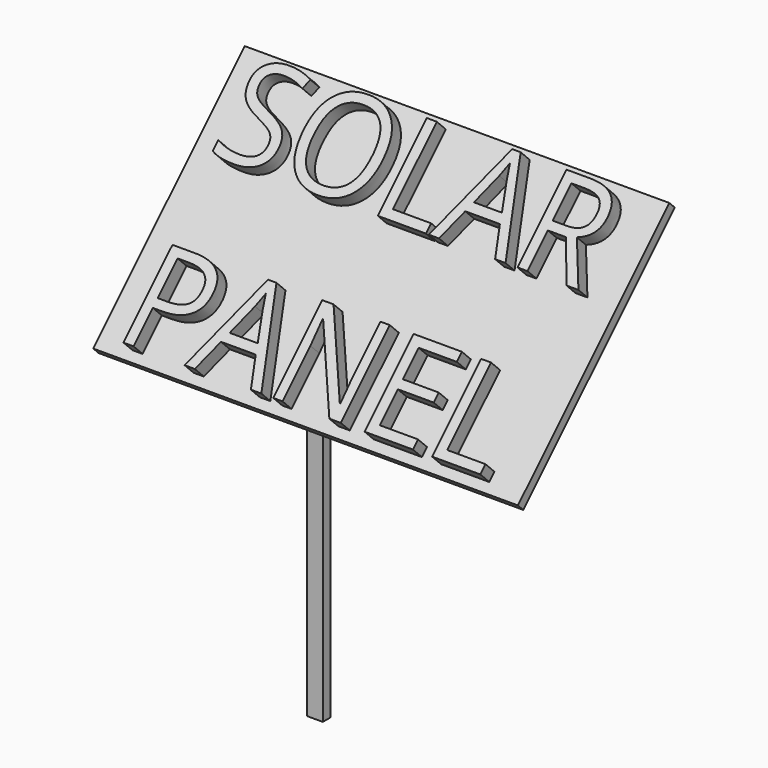
from build123d import *

# Parameters (mm, degrees)
F0_W         = 25
F0_H         = 396.1333930492
F1_DEPTH     = 15
F2_W         = 668.0434644222
F2_H         = 421.1661219597
F3_DEPTH     = 15
F4_TEXT_SIZE = 190.7505836769
F5_DEPTH     = 25
F6_ANGLE     = 45


# Not quite as in the source:
# - Text() gives the source's letters only with a copy of the font that has no kerning and outlines rounded to 1/6400 em; it was checked with that copy


with BuildPart() as f1:
    # F0 (on Front) → F1 (new body)
    with BuildSketch(Plane.XZ):
        with Locations((12.5, 198.0666965246)):
            Rectangle(F0_W, F0_H)
    extrude(amount=-F1_DEPTH)


with BuildPart() as f3:
    # F2 (on face) → F3 (new body)
    with BuildSketch(Plane.XY.offset(396.1333930492)):
        with Locations((6.4331740141, 210.5830609798)):
            Rectangle(F2_W, F2_H)
    extrude(amount=F3_DEPTH)

    # F4 (on face) → F5 (join)
    with BuildSketch(Plane.XY.offset(411.1333930492)):
        with Locations((-293.1137440627, 274.5015989388)):
            Text('SOLAR', F4_TEXT_SIZE, font='Open Sans', text_align=(TextAlign.LEFT, TextAlign.BOTTOM))
        with Locations((-293.1137440627, 15.0808051382)):
            Text('PANEL', F4_TEXT_SIZE, font='Open Sans', text_align=(TextAlign.LEFT, TextAlign.BOTTOM))
    extrude(amount=F5_DEPTH)


with BuildPart() as f3_1:
    # F6: moved
    add(f3.part.rotate(Axis((6.4331740141, 0, 396.1333930492), (1, 0, 0)), F6_ANGLE))


solid = Compound([f1.part, f3_1.part])
